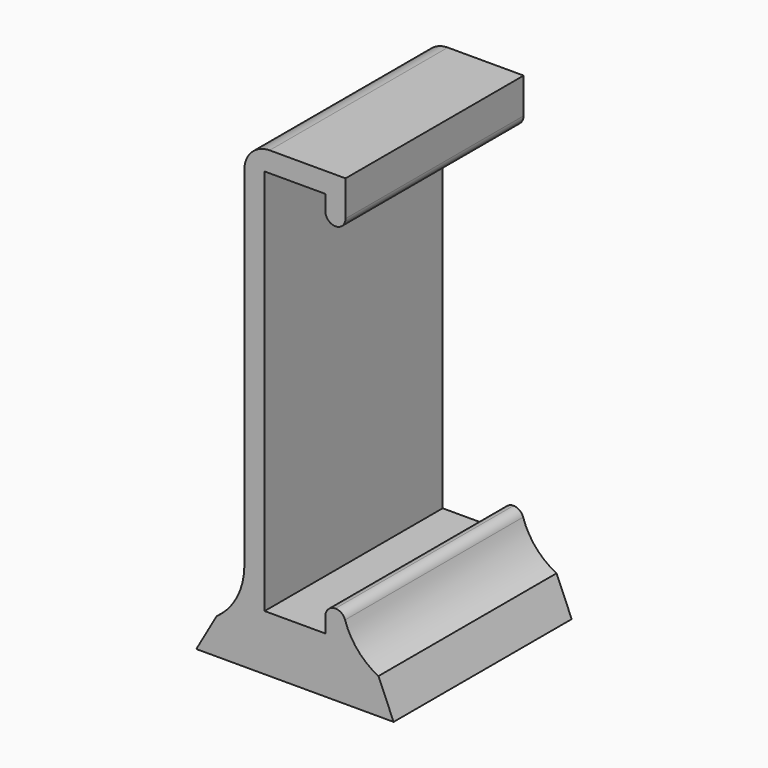
from build123d import *

# Parameters (mm, degrees)
F0_W         = 39
F0_H         = 44
F1_DEPTH     = 7
F3_DEPTH     = 44
F4_W         = 20
F4_H         = 44
F5_DEPTH     = 5
F6_W         = 20
F6_H         = 44
F7_DEPTH     = 79.5
F8_W         = 12
F8_H         = 76.5
F9_DEPTH     = 44
F10_W        = 4
F10_H        = 66.5
F11_DEPTH    = 44
F12_R        = 1.99999
F13_T1_DEPTH = 44
F14_R        = 5


# Not quite as in the source:
# - a fillet or chamfer that OpenCascade refuses, or shapes differently, is made with other operations: its cross-section is extruded or revolved along the edge and cut away or added
# - a fillet or chamfer is up to 0.001 mm smaller than in the source, because OpenCascade refuses the exact size


with BuildPart() as f1:
    # F0 (on Top) → F1 (new body)
    with BuildSketch(Plane.XY):
        Rectangle(F0_W, F0_H)
    extrude(amount=F1_DEPTH)

    # F2 (on face) → F3 (cut)
    with BuildSketch(Plane.XZ.offset(22)):
        Polygon((-19.5, 7), (-19.5, 0), (-15.5, 7), align=None)
        Polygon((16.5, 7), (19.5, 0), (19.5, 7), align=None)
    extrude(amount=-F3_DEPTH, mode=Mode.SUBTRACT)

    # F4 (on face) → F5 (join)
    with BuildSketch(Plane.XY.offset(7)):
        Rectangle(F4_W, F4_H)
    extrude(amount=F5_DEPTH)

    # F6 (on face) → F7 (join)
    with BuildSketch(Plane.XY.offset(12)):
        Rectangle(F6_W, F6_H)
    extrude(amount=F7_DEPTH)

    # F8 (on face) → F9 (cut)
    with BuildSketch(Plane.XZ.offset(22)):
        with Locations((0, 49.25)):
            Rectangle(F8_W, F8_H)
    extrude(amount=-F9_DEPTH, mode=Mode.SUBTRACT)

    # F10 (on face) → F11 (cut)
    with BuildSketch(Plane.XZ.offset(22)):
        with Locations((8, 49.25)):
            Rectangle(F10_W, F10_H)
    extrude(amount=-F11_DEPTH, mode=Mode.SUBTRACT)

    # F12 (radius 2 in the source; OpenCascade refuses exactly that, so slightly less here)
    f12_edges = [f1.edges().sort_by_distance(p)[0] for p in [
        (10, 0, 82.5),
        (6, 0, 16),
        (10, 0, 16),
        (6, 0, 82.5),
    ]]
    fillet(f12_edges, radius=F12_R)

    # F13: fillet of radius 13 on 2 edges, made by hand

    # F13_s2 → F13_t1 (join)
    with BuildSketch(Plane.XZ.offset(-22)):
        with BuildLine():
            ThreePointArc((16.5, 7), (12.4319250008, 10.1446687277), (9.9012785359, 14.6206048393))
            Line((9.9012785359, 14.6206048393), (8.6654478084, 14.2172161768))
            ThreePointArc((8.6654478084, 14.2172161768), (8.7, 14.00001), (8.7, 7))
            Line((8.7, 7), (10, 5.7))
            ThreePointArc((10, 5.7), (13.25, 5.7), (15.9240414189, 5.8345508536))
            Line((15.9240414189, 5.8345508536), (16.5, 7))
        make_face()
        with BuildLine():
            ThreePointArc((-10, 17.6183802908), (-11.4566036194, 11.6392499192), (-15.5, 7))
            Line((-15.5, 7), (-15.35, 6.7876323942))
            ThreePointArc((-15.35, 6.7876323942), (-12.75, 6.74), (-10, 6.74))
            Line((-10, 6.74), (-9.74, 7))
            Line((-9.74, 7), (-9.74, 17.6183802908))
            Line((-9.74, 17.6183802908), (-10, 17.6183802908))
        make_face()
    extrude(amount=F13_T1_DEPTH)

    # F14
    f14_edges = [f1.edges().sort_by_distance(p)[0] for p in [
        (-10, 0, 91.5),
    ]]
    fillet(f14_edges, radius=F14_R)


solid = f1.part
